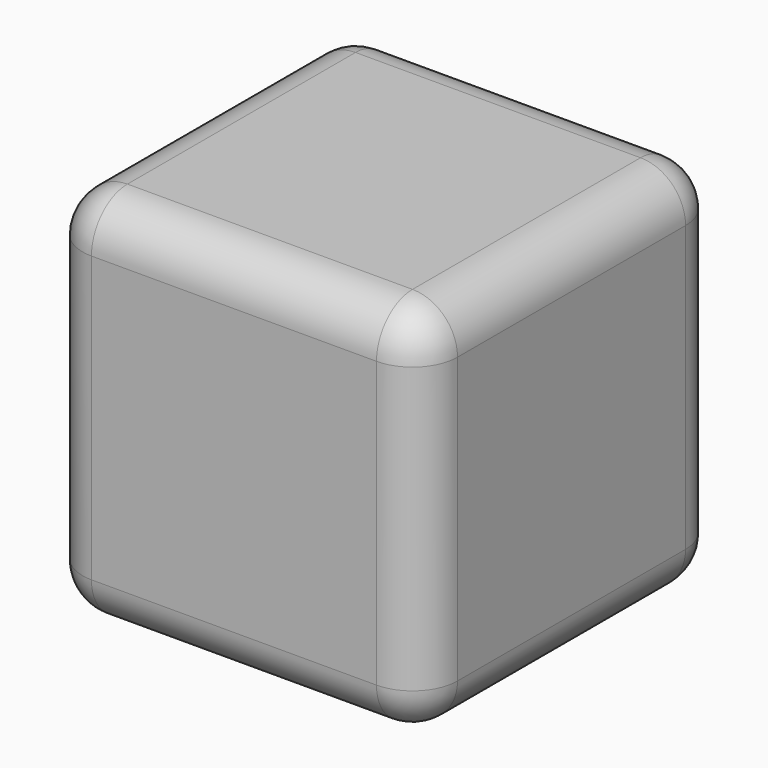
from build123d import *

# Parameters (mm, degrees)
F0_W         = 25
F0_H         = 25
F1_DEPTH     = 25
F2_R         = 3
F3_R         = 3
F4_R         = 3
F5_T1_DEPTH  = 19
F5_T3_DEPTH  = 19
F5_S7_W      = 3
F5_S7_H      = 3
F5_T8_DEPTH  = 3
F5_S13_W     = 3
F5_S13_H     = 3
F5_T14_DEPTH = 3
F5_T18_ANGLE = 90
F5_T20_ANGLE = 90


# Not quite as in the source:
# - a fillet or chamfer that OpenCascade refuses, or shapes differently, is made with other operations: its cross-section is extruded or revolved along the edge and cut away or added


with BuildPart() as f1:
    # F0 (on Front) → F1 (new body)
    with BuildSketch(Plane.XZ):
        with Locations((-12.5, 12.5)):
            Rectangle(F0_W, F0_H)
    extrude(amount=F1_DEPTH)

    # F2
    f2_edges = [f1.edges().sort_by_distance(p)[0] for p in [
        (0, -12.5, 0),
    ]]
    fillet(f2_edges, radius=F2_R)

    # F3
    f3_edges = [f1.edges().sort_by_distance(p)[0] for p in [
        (-25, -12.5, 0),
        (-14, -25, 0),
        (-25, -25, 12.5),
    ]]
    fillet(f3_edges, radius=F3_R)

    # F4
    f4_edges = [f1.edges().sort_by_distance(p)[0] for p in [
        (-12.5, 0, 0),
        (0, 0, 14),
        (-25, 0, 14),
        (-12.5, 0, 25),
    ]]
    fillet(f4_edges, radius=F4_R)

    # F5: fillet of radius 3 on 3 edges, made by hand

    # F5_s2 → F5_t1 (cut)
    with BuildSketch(Plane.XZ.offset(3)):
        with BuildLine():
            ThreePointArc((-25, 22), (-24.1213203436, 24.1213203436), (-22, 25))
            Line((-22, 25), (-25, 25))
            Line((-25, 25), (-25, 22))
        make_face()
        with BuildLine():
            ThreePointArc((0, 22), (-0.8786796564, 24.1213203436), (-3, 25))
            Line((-3, 25), (0, 25))
            Line((0, 25), (0, 22))
        make_face()
    extrude(amount=F5_T1_DEPTH, mode=Mode.SUBTRACT)

    # F5_s4 → F5_t3 (cut)
    with BuildSketch(Plane.YZ.offset(-22)):
        with BuildLine():
            ThreePointArc((-25, 22), (-24.1213203436, 24.1213203436), (-22, 25))
            Line((-22, 25), (-25, 25))
            Line((-25, 25), (-25, 22))
        make_face()
    extrude(amount=F5_T3_DEPTH, mode=Mode.SUBTRACT)


with BuildPart() as f5_tool6:
    # F5_s7 → F5_t8 (new body)
    with BuildSketch(Plane.YZ.offset(-3)):
        with Locations((-1.5, 23.5)):
            Rectangle(F5_S7_W, F5_S7_H)
    extrude(amount=F5_T8_DEPTH)

    # F5_s9 → F5_t10 (revolve, cut)
    with BuildSketch(Plane(origin=(-3, -3, 22), x_dir=(0, -0.7071067812, -0.7071067812), z_dir=(0, -0.7071067812, 0.7071067812))):
        with BuildLine():
            ThreePointArc((0, -3), (3, 0), (0, 3))
            Line((0, 3), (0, -3))
        make_face()
    revolve(axis=Axis((-3, -3, 22), (1, 0, 0)), mode=Mode.SUBTRACT)


with BuildPart() as f1_1:
    add(f1.part)

    # F5_t5: cut F5_tool6
    add(f5_tool6.part, mode=Mode.SUBTRACT)


with BuildPart() as f5_tool12:
    # F5_s13 → F5_t14 (new body)
    with BuildSketch(Plane.YZ.offset(-22)):
        with Locations((-1.5, 23.5)):
            Rectangle(F5_S13_W, F5_S13_H)
    extrude(amount=-F5_T14_DEPTH)

    # F5_s15 → F5_t16 (revolve, cut)
    with BuildSketch(Plane(origin=(-22, -3, 22), x_dir=(0, -0.7071067812, -0.7071067812), z_dir=(0, 0.7071067812, -0.7071067812))):
        with BuildLine():
            ThreePointArc((0, -3), (3, 0), (0, 3))
            Line((0, 3), (0, -3))
        make_face()
    revolve(axis=Axis((-22, -3, 22), (-1, 0, 0)), mode=Mode.SUBTRACT)


with BuildPart() as f1_2:
    add(f1_1.part)

    # F5_t11: cut F5_tool12
    add(f5_tool12.part, mode=Mode.SUBTRACT)

    # F5_s17 → F5_t18 (revolve, cut)
    with BuildSketch(Plane.XZ.offset(22)):
        with BuildLine():
            ThreePointArc((-3, 25), (-0.8786796564, 24.1213203436), (0, 22))
            Line((0, 22), (0, 25))
            Line((0, 25), (-3, 25))
        make_face()
    revolve(axis=Axis((-3, -22, 25), (0, 0, -1)), revolution_arc=F5_T18_ANGLE, mode=Mode.SUBTRACT)

    # F5_s19 → F5_t20 (revolve, cut)
    with BuildSketch(Plane.XZ.offset(22)):
        with BuildLine():
            ThreePointArc((-25, 22), (-24.1213203436, 24.1213203436), (-22, 25))
            Line((-22, 25), (-25, 25))
            Line((-25, 25), (-25, 22))
        make_face()
    revolve(axis=Axis((-22, -22, 25), (0, 0, 1)), revolution_arc=F5_T20_ANGLE, mode=Mode.SUBTRACT)


solid = f1_2.part
